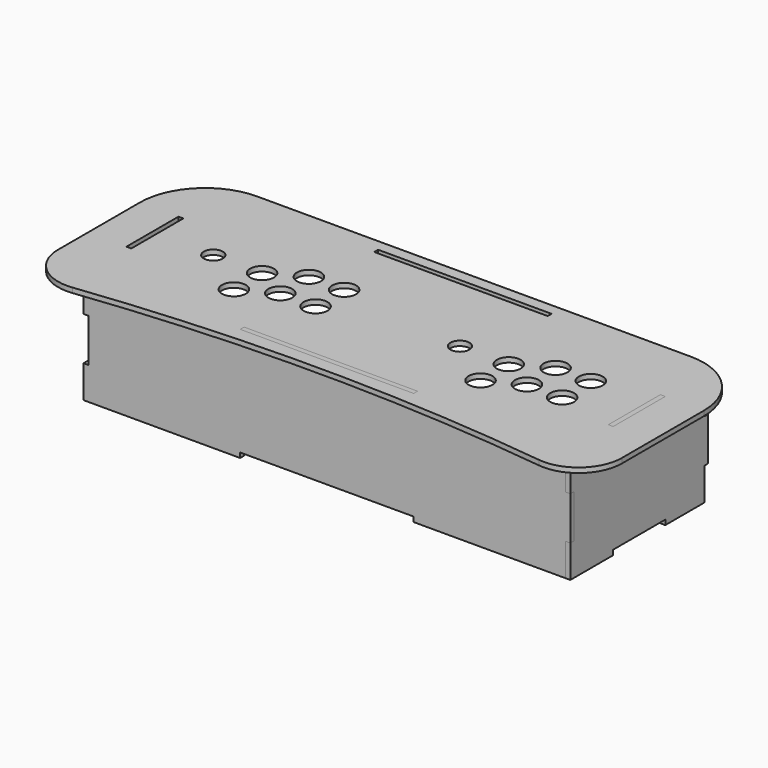
from build123d import *

# Parameters (mm, degrees)
F0_W      = 660.4
F0_H      = 254
F1_DEPTH  = 5.715
F3_DEPTH  = 5.716
F5_R      = 50.8
F6_R      = 11.1125
F6_R_2    = 14
F7_DEPTH  = 5.716
F8_R      = 76.2
F12_DEPTH = 5.715
F14_W     = 5.715
F14_H     = 38.1037298436
F14_W_2   = 76.2
F14_H_2   = 5.715
F14_H_3   = 38.1
F15_DEPTH = 5.715
F16_W     = 203.2
F16_H     = 5.715
F16_W_2   = 5.715
F16_H_2   = 76.2
F17_DEPTH = 25.4


with BuildPart() as f1:
    # F0 (on Top) → F1 (new body)
    with BuildSketch(Plane.XY):
        Rectangle(F0_W, F0_H)
    extrude(amount=F1_DEPTH)

    # F2 (on face) → F3 (cut, through all)
    with BuildSketch(Plane.XY.offset(5.715)):
        with BuildLine():
            Line((-330.2, -127), (330.2, -127))
            ThreePointArc((330.2, -127), (0, -103.0265162018), (-330.2, -127))
        make_face()
    extrude(amount=-F3_DEPTH, mode=Mode.SUBTRACT)

    # F5
    f5_edges = [f1.edges().sort_by_distance(p)[0] for p in [
        (-330.2, -127, 2.8575),
        (330.2, -127, 2.8575),
    ]]
    fillet(f5_edges, radius=F5_R)

    # F6 (on face) → F7 (cut, through all)
    with BuildSketch(Plane.XY.offset(5.715)):
        with Locations((-212.725, 11.2734837982)):
            Circle(F6_R)
        with Locations((76.2, 11.2734837982)):
            Circle(F6_R)
        with Locations((-117.475, 32.2284837982)):
            Circle(F6_R_2)
        with Locations((-117.475, -9.6815162018)):
            Circle(F6_R_2)
        with Locations((-155.575, 11.2734837982)):
            Circle(F6_R_2)
        with Locations((-155.575, -30.0015162018)):
            Circle(F6_R_2)
        with Locations((-76.2, -9.6815162018)):
            Circle(F6_R_2)
        with Locations((-76.2, 32.2284837982)):
            Circle(F6_R_2)
        with Locations((171.45, 32.2284837982)):
            Circle(F6_R_2)
        with Locations((212.725, 32.2284837982)):
            Circle(F6_R_2)
        with Locations((212.725, -9.6815162018)):
            Circle(F6_R_2)
        with Locations((171.45, -9.6815162018)):
            Circle(F6_R_2)
        with Locations((133.35, 11.2734837982)):
            Circle(F6_R_2)
        with Locations((133.35, -30.0015162018)):
            Circle(F6_R_2)
    extrude(amount=-F7_DEPTH, mode=Mode.SUBTRACT)

    # F8
    f8_edges = [f1.edges().sort_by_distance(p)[0] for p in [
        (-330.2, 127, 2.8575),
        (330.2, 127, 2.8575),
    ]]
    fillet(f8_edges, radius=F8_R)

    # F16 (on face) → F17 (cut)
    with BuildSketch(Plane.XY.offset(5.715)):
        with Locations((0, -85.4075)):
            Rectangle(F16_W, F16_H)
        with Locations((0, 110.8075)):
            Rectangle(F16_W, F16_H)
        with Locations((282.2575, 12.7)):
            Rectangle(F16_W_2, F16_H_2)
        with Locations((-282.2575, 12.7)):
            Rectangle(F16_W_2, F16_H_2)
    extrude(amount=-F17_DEPTH, mode=Mode.SUBTRACT)


with BuildPart() as f12:
    # F11 (on offset) → F12 (new body)
    with BuildSketch(Plane.XZ.offset(82.55)):
        Polygon((-285.115, -127), (-279.4, -126.9962701564), (-101.6, -126.9962701564), (-101.6, -121.2812701564), (101.6, -121.2812701564), (101.6, -126.9962701564), (279.4, -126.9962701564), (279.4, -88.8962701564), (285.115, -88.8962701564), (285.115, -38.1), (279.4, -38.1), (279.4, 0), (101.6, 0), (101.6, 5.715), (-101.6, 5.715), (-101.6, 0), (-279.4, 0), (-285.115, 0), (-285.115, -38.1), (-279.4, -38.1), (-279.4, -88.9), (-285.115, -88.9), align=None)
    extrude(amount=F12_DEPTH)


with BuildPart() as f15:
    # F14 (on offset) → F15 (new body)
    with BuildSketch(Plane.YZ.offset(279.4)):
        Polygon((50.8, -127), (107.95, -127), (107.95, -88.9), (113.665, -88.9), (113.665, -38.1), (107.95, -38.1), (107.95, 0), (50.8, 0), (-25.4, 0), (-82.55, 0), (-82.55, -38.1), (-82.55, -88.8962701564), (-82.55, -127), (-25.4, -127), (-25.4, -121.285), (50.8, -121.285), align=None)
        with Locations((-85.4075, -107.9481350782)):
            Rectangle(F14_W, F14_H)
        with Locations((12.7, 2.8575)):
            Rectangle(F14_W_2, F14_H_2)
        with Locations((-85.4075, -19.05)):
            Rectangle(F14_W, F14_H_3)
    extrude(amount=F15_DEPTH)


solid = Compound([f1.part, f12.part, f15.part])
